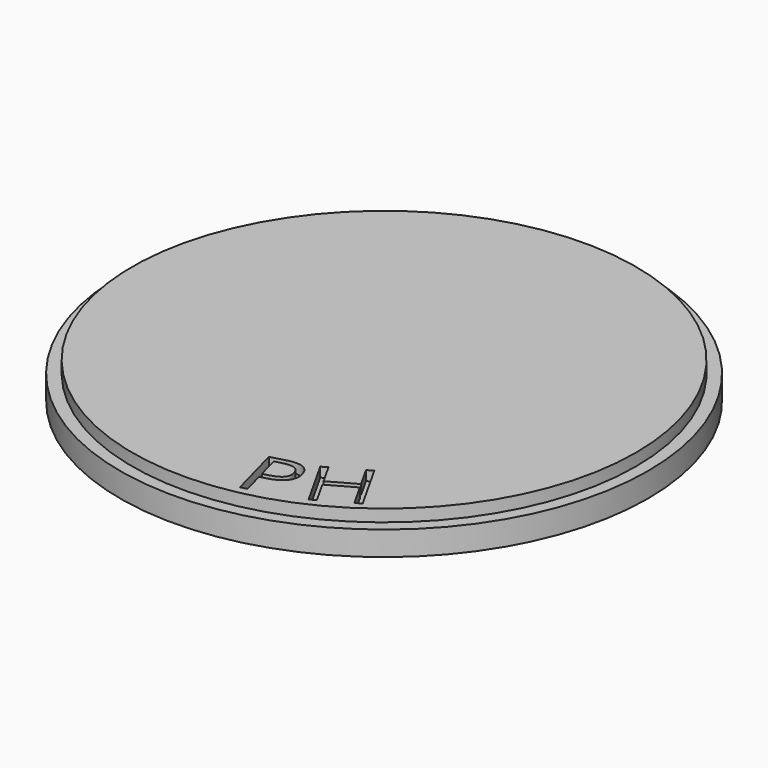
from build123d import *

# Parameters (mm, degrees)
F0_R           = 54.3578767205
F1_DEPTH       = 5
F2_T           = -2.5
F3_TEXT_SIZE   = 16.25
F3_TEXT_SIZE_2 = 16.2436548223
F4_DEPTH       = 3
F5_DEPTH       = 5


# Not quite as in the source:
# - Text() gives the source's letters only with a copy of the font that has no kerning and outlines rounded to 1/6400 em; it was checked with that copy


with BuildPart() as f1:
    # F0 (on Top) → F1 (new body)
    with BuildSketch(Plane.XY):
        Circle(F0_R)
    extrude(amount=F1_DEPTH)

    # F2
    f2_openings = [f1.faces().sort_by_distance(p)[0] for p in [
        (0, 0, 5),
    ]]
    offset(amount=F2_T, openings=f2_openings)

    # F3 (on face) → F4 (join)
    with BuildSketch(Plane.XY.offset(2.5)):
        with Locations(Location((19.5427485531, -46.377714422), (0, 0, 29.3851525555))):
            Text('H', F3_TEXT_SIZE, font='Open Sans', text_align=(TextAlign.LEFT, TextAlign.BOTTOM))
        with Locations(Location((8.1113231237, -49.59038654), (0, 0, 15))):
            Text('P', F3_TEXT_SIZE_2, font='Open Sans', text_align=(TextAlign.LEFT, TextAlign.BOTTOM))
    extrude(amount=F4_DEPTH)

    # F5 (add): faces of the model
    f5_faces = [f1.faces().sort_by_distance(p)[0] for p in [
        (-0.1702309022, 0.4315272611, 2.5),
        (10.8844026816, -40.4754565505, 2.5),
    ]]
    extrude(f5_faces, amount=F5_DEPTH)


solid = f1.part
